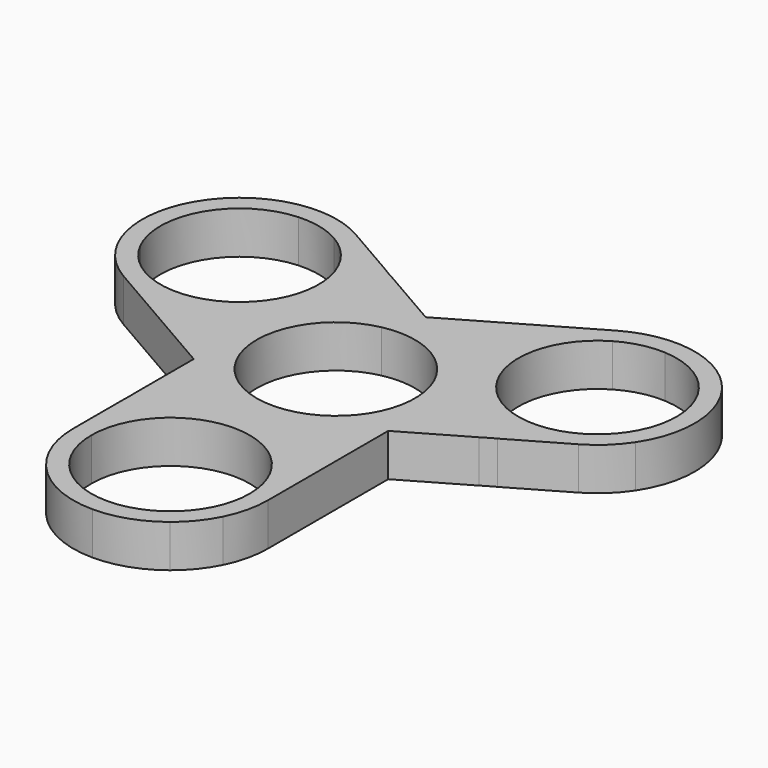
from build123d import *

# Parameters (mm, degrees)
F1_DEPTH        = 7
F1_COPIES_COUNT = 3


# Not quite as in the source:
# - a feature of the source that left no trace in its solid (it failed there, or was rolled back) is left out
# - a pattern or mirror of a feature is missing from the dataset's text; its kind, count and spacing are read off the source's solid


with BuildPart() as f1:
    # F0 (on Top) → F1 (new body)
    with BuildSketch(Plane.XY):
        with BuildLine():
            Line((0.1390978545, -12.9589841303), (0.1390978545, 21.0410158697))
            ThreePointArc((0.1390978545, 21.0410158697), (-15.8609021455, 5.0410158697), (-31.8609021455, 21.0410158697))
            Line((-31.8609021455, 21.0410158697), (-31.8609021455, 0))
            ThreePointArc((-31.8609021455, 0), (-31.8301791681, -1.1947273097), (-31.8609021455, -2.3894546193))
            Line((-31.8609021455, -2.3894546193), (-31.8609021455, -12.9589841303))
            ThreePointArc((-31.8609021455, -12.9589841303), (-15.8609021455, 3.0410158697), (0.1390978545, -12.9589841303))
        make_face()
        with BuildLine():
            Line((0.1390978545, 21.0410158697), (-2.8359021455, 21.0410158697))
            ThreePointArc((-2.8359021455, 21.0410158697), (-15.8609021455, 8.0160158697), (-28.8859021455, 21.0410158697))
            Line((-28.8859021455, 21.0410158697), (-31.8609021455, 21.0410158697))
            ThreePointArc((-31.8609021455, 21.0410158697), (-15.8609021455, 5.0410158697), (0.1390978545, 21.0410158697))
        make_face()
        with BuildLine():
            ThreePointArc((-28.8859021455, 21.0410158697), (-15.8609021455, 34.0660158697), (-2.8359021455, 21.0410158697))
            Line((-2.8359021455, 21.0410158697), (0.1390978545, 21.0410158697))
            ThreePointArc((0.1390978545, 21.0410158697), (-15.8609021455, 37.0410158697), (-31.8609021455, 21.0410158697))
            Line((-31.8609021455, 21.0410158697), (-28.8859021455, 21.0410158697))
        make_face()
        with BuildLine():
            Line((-2.8359021455, -12.9589841303), (0.1390978545, -12.9589841303))
            ThreePointArc((0.1390978545, -12.9589841303), (-15.8609021455, 3.0410158697), (-31.8609021455, -12.9589841303))
            Line((-31.8609021455, -12.9589841303), (-28.8859021455, -12.9589841303))
            ThreePointArc((-28.8859021455, -12.9589841303), (-15.8609021455, 0.0660158697), (-2.8359021455, -12.9589841303))
        make_face()
        with BuildLine():
            Line((-28.8859021455, -12.9589841303), (-31.8609021455, -12.9589841303))
            ThreePointArc((-31.8609021455, -12.9589841303), (-31.4346103213, -16.6277187425), (-30.1784504386, -20.1009594084))
            Line((-30.1784504386, -20.1009594084), (-26.7532303689, -20.1009594084))
            ThreePointArc((-26.7532303689, -20.1009594084), (-28.3413508576, -16.6857823466), (-28.8859021455, -12.9589841303))
        make_face()
        with BuildLine():
            ThreePointArc((-1.5433538524, -20.1009594084), (-0.2871939697, -16.6277187425), (0.1390978545, -12.9589841303))
            Line((0.1390978545, -12.9589841303), (-2.8359021455, -12.9589841303))
            ThreePointArc((-2.8359021455, -12.9589841303), (-3.3804534334, -16.6857823466), (-4.9685739221, -20.1009594084))
            Line((-4.9685739221, -20.1009594084), (-1.5433538524, -20.1009594084))
        make_face()
        with BuildLine():
            ThreePointArc((-5.9366183214, -25.5092267804), (-3.4420074647, -23.0471482302), (-1.5433538524, -20.1009594084))
            Line((-1.5433538524, -20.1009594084), (-4.9685739221, -20.1009594084))
            ThreePointArc((-4.9685739221, -20.1009594084), (-15.8609021455, -25.9839841303), (-26.7532303689, -20.1009594084))
            Line((-26.7532303689, -20.1009594084), (-30.1784504386, -20.1009594084))
            ThreePointArc((-30.1784504386, -20.1009594084), (-24.2789897171, -26.5654458906), (-15.8609022277, -28.9589841303))
            ThreePointArc((-15.8609022277, -28.9589841303), (-10.6075167236, -28.0719567567), (-5.9366183214, -25.5092267804))
        make_face()
    extrude(amount=F1_DEPTH)

    # F1_copies: F1 ×3 about axis
    f1_copies_axis = Axis((-15.860902, 21.041016, 0), (0, 0, 1))


with BuildPart() as f1_1:
    add(f1.part)
    for i in range(1, F1_COPIES_COUNT):
        add(f1.part.rotate(f1_copies_axis, i * 360 / F1_COPIES_COUNT))


solid = f1_1.part
